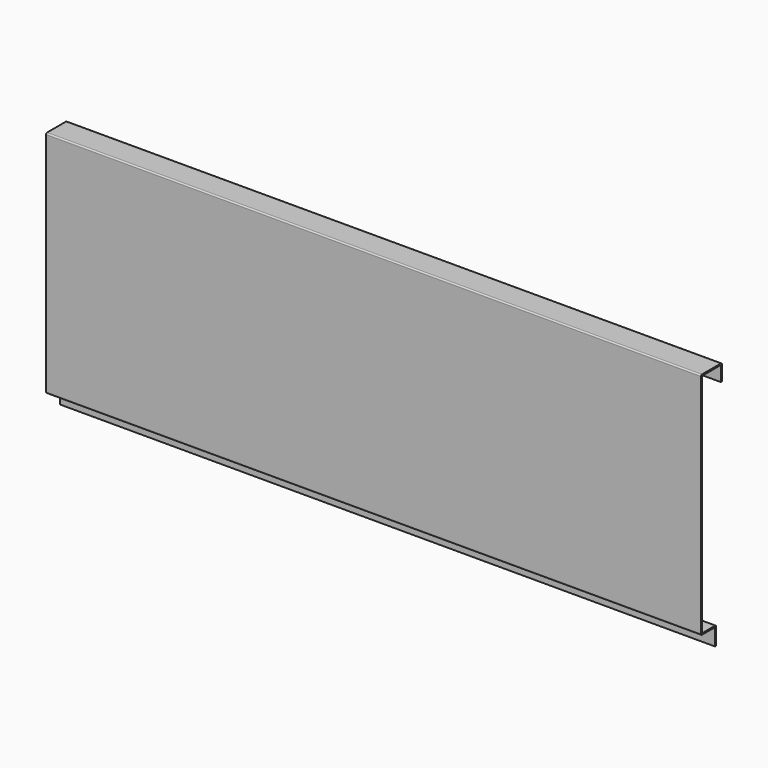
from build123d import *

# Parameters (mm, degrees)
F1_DEPTH = 1000
F3_D     = 8
F4_R     = 2


# Not quite as in the source:
# - a feature names something its author has since deleted; it is built from what else it names


with BuildPart() as f1:
    # F0 (on Right) → F1 (new body)
    with BuildSketch(Plane.YZ):
        Polygon((-18.8378913403, 427.8021101952), (-18.8378913403, 404.8021101952), (-16.8378913403, 404.8021101952), (-16.8378913403, 429.8021101952), (-56.8378913403, 429.8021101952), (-56.8378913403, 79.8021101952), (-29.8378913403, 79.8021101952), (-29.8378913403, 53.8021101952), (-27.8378913403, 53.8021101952), (-27.8378913403, 81.8021101952), (-54.8378913403, 81.8021101952), (-54.8378913403, 427.8021101952), align=None)
    extrude(amount=F1_DEPTH)

    # F3 (through all)
    with Locations(Plane.XZ.offset(29.8378913403)):
        with Locations((350, 66.8021101952), (650, 66.8021101952), (900, 66.8021101952), (100, 66.8021101952)):
            Hole(F3_D / 2)

    # F4
    f4_edges = [f1.edges().sort_by_distance(p)[0] for p in [
        (500, -56.837891, 429.80211),
        (500, -16.837891, 429.80211),
        (500, -56.837891, 79.80211),
        (500, -27.837891, 81.80211),
        (500, -54.837891, 81.80211),
        (500, -29.837891, 79.80211),
        (500, -18.837891, 427.80211),
        (500, -54.837891, 427.80211),
    ]]
    fillet(f4_edges, radius=F4_R)


solid = f1.part
